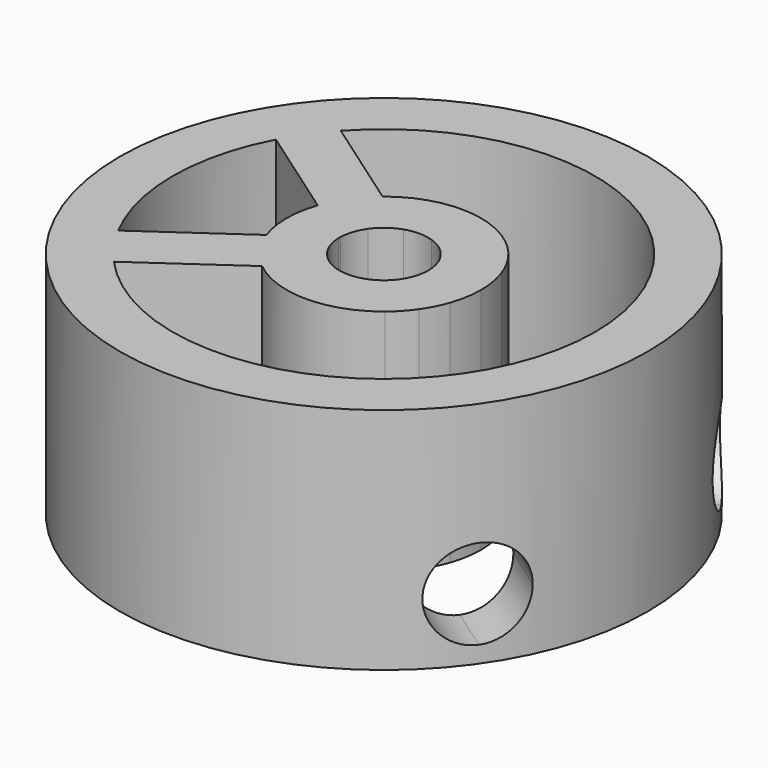
from build123d import *

# Parameters (mm, degrees)
F0_R     = 30
F0_R_2   = 24
F1_DEPTH = 26
F3_DEPTH = 26
F7_START = -13.9
F7_DEPTH = 10.2
F8_R     = 5.099


# Not quite as in the source:
# - a fillet or chamfer is up to 0.001 mm smaller than in the source, because OpenCascade refuses the exact size


with BuildPart() as f1:
    # F0 (on Top) → F1 (new body)
    with BuildSketch(Plane.XY):
        Circle(F0_R)
        Circle(F0_R_2, mode=Mode.SUBTRACT)
    extrude(amount=F1_DEPTH)

    # F2 (on face) → F3 (join)
    with BuildSketch(Plane.XY.offset(26)):
        with BuildLine():
            ThreePointArc((-10.4323833788, 3.642509717), (-9.8347922509, 5.0377933048), (-9.0516300894, 6.3380196217))
            Line((-9.0516300894, 6.3380196217), (-19.6596490629, 13.7658344724))
            ThreePointArc((-19.6596490629, 13.7658344724), (-20.4831189166, 12.5076712241), (-21.2261826653, 11.2004093434))
            Line((-21.2261826653, 11.2004093434), (-10.4323833788, 3.642509717))
        make_face()
        with BuildLine():
            ThreePointArc((-9.0516300894, 6.3380196217), (-8.0976742488, 7.518654917), (-6.9909247607, 8.5574219828))
            Line((-6.9909247607, 8.5574219828), (-17.7847240472, 16.1153216091))
            ThreePointArc((-17.7847240472, 16.1153216091), (-18.7590056201, 14.9699601919), (-19.6596490629, 13.7658344724))
            Line((-19.6596490629, 13.7658344724), (-9.0516300894, 6.3380196217))
        make_face()
        with BuildLine():
            ThreePointArc((-4.1367178237, 2.8965610036), (-3.0234595129, 4.044897103), (-1.6069340915, 4.7875111306))
            Line((-1.6069340915, 4.7875111306), (-6.9909247607, 8.5574219828))
            ThreePointArc((-6.9909247607, 8.5574219828), (-8.0976742488, 7.518654917), (-9.0516300894, 6.3380196217))
            Line((-9.0516300894, 6.3380196217), (-4.1367178237, 2.8965610036))
        make_face()
        with BuildLine():
            ThreePointArc((-5.0483927096, 0.1274011352), (-4.7967307066, 1.5792005979), (-4.1367178237, 2.8965610036))
            Line((-4.1367178237, 2.8965610036), (-9.0516300894, 6.3380196217))
            ThreePointArc((-9.0516300894, 6.3380196217), (-9.8347922509, 5.0377933048), (-10.4323833788, 3.642509717))
            Line((-10.4323833788, 3.642509717), (-5.2303403869, 0))
            Line((-5.2303403869, 0), (-5.0483927096, 0.1274011352))
        make_face()
        with BuildLine():
            Line((-10.4323833788, -3.642509717), (-5.2303403869, 0))
            Line((-5.2303403869, 0), (-10.4323833788, 3.642509717))
            ThreePointArc((-10.4323833788, 3.642509717), (-11.05, 0), (-10.4323833788, -3.642509717))
        make_face()
        with BuildLine():
            Line((-9.0516300894, -6.3380196217), (-4.1367178237, -2.8965610036))
            ThreePointArc((-4.1367178237, -2.8965610036), (-4.7967307066, -1.5792005979), (-5.0483927096, -0.1274011352))
            Line((-5.0483927096, -0.1274011352), (-5.2303403869, 0))
            Line((-5.2303403869, 0), (-10.4323833788, -3.642509717))
            ThreePointArc((-10.4323833788, -3.642509717), (-9.8347922509, -5.0377933048), (-9.0516300894, -6.3380196217))
        make_face()
        with BuildLine():
            Line((-6.9909247607, -8.5574219828), (-1.6069340915, -4.7875111306))
            ThreePointArc((-1.6069340915, -4.7875111306), (-3.0234595129, -4.044897103), (-4.1367178237, -2.8965610036))
            Line((-4.1367178237, -2.8965610036), (-9.0516300894, -6.3380196217))
            ThreePointArc((-9.0516300894, -6.3380196217), (-8.0976742488, -7.518654917), (-6.9909247607, -8.5574219828))
        make_face()
        with BuildLine():
            Line((6.9909247607, -8.5574219828), (1.6069340915, -4.7875111306))
            ThreePointArc((1.6069340915, -4.7875111306), (0, -5.05), (-1.6069340915, -4.7875111306))
            Line((-1.6069340915, -4.7875111306), (-6.9909247607, -8.5574219828))
            ThreePointArc((-6.9909247607, -8.5574219828), (0, -11.05), (6.9909247607, -8.5574219828))
        make_face()
        with BuildLine():
            Line((9.0516300894, -6.3380196217), (4.1367178237, -2.8965610036))
            ThreePointArc((4.1367178237, -2.8965610036), (3.0234595129, -4.044897103), (1.6069340915, -4.7875111306))
            Line((1.6069340915, -4.7875111306), (6.9909247607, -8.5574219828))
            ThreePointArc((6.9909247607, -8.5574219828), (8.0976742488, -7.518654917), (9.0516300894, -6.3380196217))
        make_face()
        with BuildLine():
            Line((5.2303403869, 0), (5.0483927096, -0.1274011352))
            ThreePointArc((5.0483927096, -0.1274011352), (4.7967307066, -1.5792005979), (4.1367178237, -2.8965610036))
            Line((4.1367178237, -2.8965610036), (9.0516300894, -6.3380196217))
            ThreePointArc((9.0516300894, -6.3380196217), (9.8347922509, -5.0377933048), (10.4323833788, -3.642509717))
            Line((10.4323833788, -3.642509717), (5.2303403869, 0))
        make_face()
        with BuildLine():
            Line((10.4323833788, 3.642509717), (5.2303403869, 0))
            Line((5.2303403869, 0), (10.4323833788, -3.642509717))
            ThreePointArc((10.4323833788, -3.642509717), (10.8945017402, -1.8472498024), (11.05, 0))
            ThreePointArc((11.05, 0), (10.8945017402, 1.8472498024), (10.4323833788, 3.642509717))
        make_face()
        with BuildLine():
            ThreePointArc((4.1367178237, 2.8965610036), (4.7967307066, 1.5792005979), (5.0483927096, 0.1274011352))
            Line((5.0483927096, 0.1274011352), (5.2303403869, 0))
            Line((5.2303403869, 0), (10.4323833788, 3.642509717))
            ThreePointArc((10.4323833788, 3.642509717), (9.8347922509, 5.0377933048), (9.0516300894, 6.3380196217))
            Line((9.0516300894, 6.3380196217), (4.1367178237, 2.8965610036))
        make_face()
        with BuildLine():
            ThreePointArc((1.6069340915, 4.7875111306), (3.0234595129, 4.044897103), (4.1367178237, 2.8965610036))
            Line((4.1367178237, 2.8965610036), (9.0516300894, 6.3380196217))
            ThreePointArc((9.0516300894, 6.3380196217), (8.0976742488, 7.518654917), (6.9909247607, 8.5574219828))
            Line((6.9909247607, 8.5574219828), (1.6069340915, 4.7875111306))
        make_face()
        with BuildLine():
            ThreePointArc((-1.6069340915, 4.7875111306), (0, 5.05), (1.6069340915, 4.7875111306))
            Line((1.6069340915, 4.7875111306), (6.9909247607, 8.5574219828))
            ThreePointArc((6.9909247607, 8.5574219828), (0, 11.05), (-6.9909247607, 8.5574219828))
            Line((-6.9909247607, 8.5574219828), (-1.6069340915, 4.7875111306))
        make_face()
        with BuildLine():
            ThreePointArc((-5.0483927096, -0.1274011352), (-5.05, 0), (-5.0483927096, 0.1274011352))
            Line((-5.0483927096, 0.1274011352), (-5.2303403869, 0))
            Line((-5.2303403869, 0), (-5.0483927096, -0.1274011352))
        make_face()
        with BuildLine():
            ThreePointArc((5.0483927096, 0.1274011352), (5.0495981614, 0.0637056368), (5.05, 0))
            ThreePointArc((5.05, 0), (5.0495981614, -0.0637056368), (5.0483927096, -0.1274011352))
            Line((5.0483927096, -0.1274011352), (5.2303403869, 0))
            Line((5.2303403869, 0), (5.0483927096, 0.1274011352))
        make_face()
        with BuildLine():
            Line((-19.6596490629, -13.7658344724), (-9.0516300894, -6.3380196217))
            ThreePointArc((-9.0516300894, -6.3380196217), (-9.8347922509, -5.0377933048), (-10.4323833788, -3.642509717))
            Line((-10.4323833788, -3.642509717), (-21.2261826653, -11.2004093434))
            ThreePointArc((-21.2261826653, -11.2004093434), (-20.4831189166, -12.5076712241), (-19.6596490629, -13.7658344724))
        make_face()
        with BuildLine():
            Line((-17.7847240472, -16.1153216091), (-6.9909247607, -8.5574219828))
            ThreePointArc((-6.9909247607, -8.5574219828), (-8.0976742488, -7.518654917), (-9.0516300894, -6.3380196217))
            Line((-9.0516300894, -6.3380196217), (-19.6596490629, -13.7658344724))
            ThreePointArc((-19.6596490629, -13.7658344724), (-18.7590056201, -14.9699601919), (-17.7847240472, -16.1153216091))
        make_face()
    extrude(amount=-F3_DEPTH)

    # F4 (on Front) → F5 (revolve, cut)
    with BuildSketch(Plane.XZ):
        with BuildLine():
            Line((-30, 15), (-30, 8.8350883268))
            Line((-30, 8.8350883268), (-9.4916700442, 23.1951755579))
            ThreePointArc((-9.4916700442, 23.1951755579), (-12.7514645707, 25.271893707), (-16.5249488714, 24.435332378))
            Line((-16.5249488714, 24.435332378), (-30, 15))
        make_face()
        Polygon((-38.8382538388, 2.6464763642), (-30, 8.8350883268), (-30, 15), (-41.7348148424, 6.7831941879), align=None)
    revolve(axis=Axis((-24.1649619415, 0, 12.9208259611), (-0.8191520443, 0, -0.5735764364)), mode=Mode.SUBTRACT)

    # F6 (on face) → F7 (cut)
    with BuildSketch(Plane.XY.offset(26).offset(F7_START)):
        with BuildLine():
            ThreePointArc((16.2854038211, 17.629112921), (18.0760321089, 15.787877096), (19.6596490629, 13.7658344724))
            Line((19.6596490629, 13.7658344724), (24.5745613287, 17.2072930905))
            ThreePointArc((24.5745613287, 17.2072930905), (23.0169999839, 19.2410423767), (21.2916157205, 21.1345002309))
            Line((21.2916157205, 21.1345002309), (16.2854038211, 17.629112921))
        make_face()
        with BuildLine():
            Line((24.5745613287, 17.2072930905), (19.6596490629, 13.7658344724))
            ThreePointArc((19.6596490629, 13.7658344724), (21.0181186976, 11.5861419987), (22.1358834719, 9.2737620693))
            Line((22.1358834719, 9.2737620693), (27.1420953713, 12.7791493791))
            ThreePointArc((27.1420953713, 12.7791493791), (25.952943171, 15.0480809661), (24.5745613287, 17.2072930905))
        make_face()
        with BuildLine():
            ThreePointArc((22.1358834719, -9.2737620693), (21.0181186976, -11.5861419987), (19.6596490629, -13.7658344724))
            Line((19.6596490629, -13.7658344724), (24.5745613287, -17.2072930905))
            ThreePointArc((24.5745613287, -17.2072930905), (25.952943171, -15.0480809661), (27.1420953713, -12.7791493791))
            Line((27.1420953713, -12.7791493791), (22.1358834719, -9.2737620693))
        make_face()
        with BuildLine():
            Line((24.5745613287, -17.2072930905), (19.6596490629, -13.7658344724))
            ThreePointArc((19.6596490629, -13.7658344724), (18.0760321089, -15.787877096), (16.2854038211, -17.629112921))
            Line((16.2854038211, -17.629112921), (21.2916157205, -21.1345002309))
            ThreePointArc((21.2916157205, -21.1345002309), (23.0169999839, -19.2410423767), (24.5745613287, -17.2072930905))
        make_face()
    extrude(amount=-F7_DEPTH, mode=Mode.SUBTRACT)

    # F8 (radius 5.1 in the source; OpenCascade refuses exactly that, so slightly less here)
    f8_edges = [f1.edges().sort_by_distance(p)[0] for p in [
        (18.78851, -19.381807, 1.9),
        (18.78851, -19.381807, 12.1),
        (24.638989, -11.026456, 12.1),
        (24.638989, -11.026456, 1.9),
        (18.78851, 19.381807, 1.9),
        (18.78851, 19.381807, 12.1),
        (24.638989, 11.026456, 12.1),
        (24.638989, 11.026456, 1.9),
    ]]
    fillet(f8_edges, radius=F8_R)


solid = f1.part
